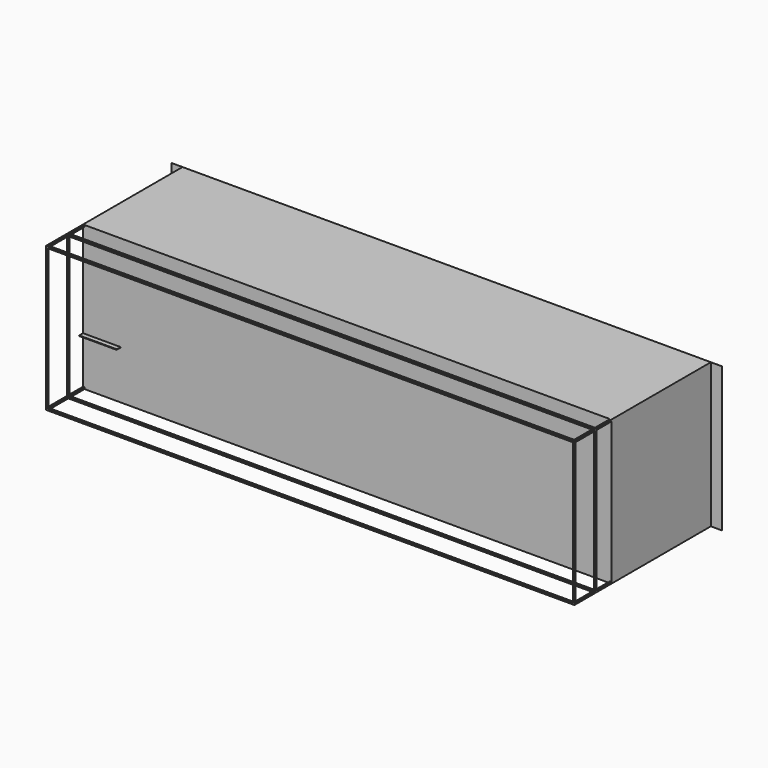
from build123d import *

# Parameters (mm, degrees)
F0_W      = 10970
F0_H      = 3000
F1_DEPTH  = 2580
F2_W      = 30
F2_H      = 2930
F3_DEPTH  = 30
F4_W      = 30
F4_H      = 35
F5_DEPTH  = 10940
F6_W      = 510
F6_H      = 2930
F7_DEPTH  = 30
F8_W      = 11430
F8_H      = 3000
F9_DEPTH  = 1
F2_W_2    = 99.7082424164
F2_H_2    = 12.0352804661
F10_DEPTH = 777


# Not quite as in the source:
# - a feature names something its author has since deleted; it is built from what else it names


with BuildPart() as f1:
    # F0 (on Front) → F1 (new body)
    with BuildSketch(Plane.XZ):
        Rectangle(F0_W, F0_H)
    extrude(amount=F1_DEPTH)

    # F2 (on face) → F3 (join)
    with BuildSketch(Plane(origin=(-5485, 0, 0), x_dir=(0, -1, 0), z_dir=(-1, 0, 0))):
        Polygon((3540, 1500), (2580, 1500), (2580, 1465), (2970, 1465), (3000, 1465), (3510, 1465), (3510, -1465), (3000, -1465), (2970, -1465), (2580, -1465), (2580, -1500), (3540, -1500), (3540, -1465), (3540, 1465), align=None)
        with Locations((2985, 0)):
            Rectangle(F2_W, F2_H)
    extrude(amount=-F3_DEPTH)

    # F4 (on face) → F5 (join)
    with BuildSketch(Plane(origin=(-5485, 0, 0), x_dir=(0, -1, 0), z_dir=(-1, 0, 0))):
        with Locations((2985, 1482.5)):
            Rectangle(F4_W, F4_H)
        with Locations((2985, -1482.5)):
            Rectangle(F4_W, F4_H)
        with Locations((3525, -1482.5)):
            Rectangle(F4_W, F4_H)
        with Locations((3525, 1482.5)):
            Rectangle(F4_W, F4_H)
    extrude(amount=-F5_DEPTH)

    # F6 (on face) → F7 (join)
    with BuildSketch(Plane.YZ.offset(5485)):
        Polygon((-3540, -1500), (-2580, -1500), (-2580, -1465), (-2969.8400497437, -1465), (-2969.8400497437, 1465), (-2580, 1465), (-2580, 1500), (-3540, 1500), (-3540, 1465), (-3540, -1465), align=None)
        with Locations((-3255, 0)):
            Rectangle(F6_W, F6_H, mode=Mode.SUBTRACT)
    extrude(amount=-F7_DEPTH)

    # F8 (on face) → F9 (join)
    with BuildSketch(Plane(origin=(0, 0, 0), x_dir=(-1, 0, 0), z_dir=(0, 1, 0))):
        Rectangle(F8_W, F8_H)
    extrude(amount=F9_DEPTH)

    # F2 (on face) → F10 (join)
    with BuildSketch(Plane(origin=(-5485, 0, 0), x_dir=(0, -1, 0), z_dir=(-1, 0, 0))):
        with Locations((2629.8541212082, -493.982359767)):
            Rectangle(F2_W_2, F2_H_2)
    extrude(amount=-F10_DEPTH)


solid = f1.part
